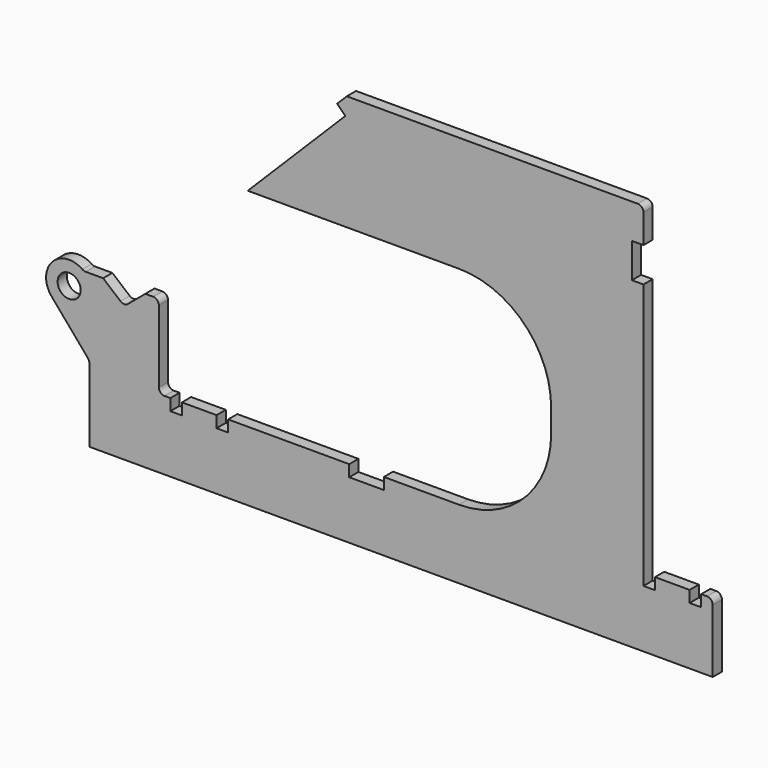
from build123d import *

# Parameters (mm, degrees)
F0_R     = 6.35
F1_DEPTH = 6.35
F2_R     = 3.175
F3_R     = 5.08
F4_R     = 3.175
F5_R     = 3.175


# Not quite as in the source:
# - ends of sketch curves that miss each other by under 0.0002 mm in the source are joined


with BuildPart() as f1:
    # F0 (on Front) → F1 (new body)
    with BuildSketch(Plane.XZ):
        with BuildLine():
            Line((-72.7094654823, -50.272475262), (-83.3648741359, -50.272475262))
            ThreePointArc((-83.3648741359, -50.272475262), (-100.4842470659, -51.222143603), (-101.056400417, -68.3582903151))
            Line((-101.056400417, -68.3582903151), (-80.147210941, -92.8018072064))
            Line((-80.147210941, -92.8018072064), (-80.147210941, -134.409975262))
            Line((-80.147210941, -134.409975262), (262.752789059, -134.409975262))
            Line((262.752789059, -134.409975262), (262.752789059, -96.309975262))
            Line((262.752789059, -96.309975262), (256.402789059, -96.309975262))
            Line((256.402789059, -96.309975262), (256.402789059, -102.659975262))
            Line((256.402789059, -102.659975262), (250.052789059, -102.659975262))
            Line((250.052789059, -102.659975262), (250.052789059, -96.309975262))
            Line((250.052789059, -96.309975262), (231.002789059, -96.309975262))
            Line((231.002789059, -96.309975262), (231.002789059, -102.659975262))
            Line((231.002789059, -102.659975262), (224.652789059, -102.659975262))
            Line((224.652789059, -102.659975262), (224.652789059, 43.390024738))
            Line((224.652789059, 43.390024738), (218.302789059, 43.390024738))
            Line((218.302789059, 43.390024738), (218.302789059, 62.440024738))
            Line((218.302789059, 62.440024738), (224.652789059, 62.440024738))
            Line((224.652789059, 62.440024738), (224.652789059, 81.490024738))
            Line((224.652789059, 81.490024738), (61.4126609984, 81.490024738))
            Line((61.4126609984, 81.490024738), (56.0792184251, 76.1565821646))
            Line((56.0792184251, 76.1565821646), (60.5693464856, 71.6664541041))
            Line((60.5693464856, 71.6664541041), (6.8929171195, 17.990024738))
            Line((6.8929171195, 17.990024738), (123.052789059, 17.990024738))
            ThreePointArc((123.052789059, 17.990024738), (158.9738135432, 3.1110492223), (173.852789059, -32.809975262))
            Line((173.852789059, -32.809975262), (173.852789059, -45.509975262))
            ThreePointArc((173.852789059, -45.509975262), (158.9738135432, -81.4309997463), (123.052789059, -96.309975262))
            Line((123.052789059, -96.309975262), (81.777789059, -96.309975262))
            Line((81.777789059, -96.309975262), (81.777789059, -102.659975262))
            Line((81.777789059, -102.659975262), (62.727789059, -102.659975262))
            Line((62.727789059, -102.659975262), (62.727789059, -96.309975262))
            Line((62.727789059, -96.309975262), (-3.947210941, -96.309975262))
            Line((-3.947210941, -96.309975262), (-3.947210941, -102.659975262))
            Line((-3.947210941, -102.659975262), (-10.297210941, -102.659975262))
            Line((-10.297210941, -102.659975262), (-10.297210941, -96.309975262))
            Line((-10.297210941, -96.309975262), (-29.347210941, -96.309975262))
            Line((-29.347210941, -96.309975262), (-29.347210941, -102.659975262))
            Line((-29.347210941, -102.659975262), (-35.697210941, -102.659975262))
            Line((-35.697210941, -102.659975262), (-35.697210941, -96.309975262))
            Line((-35.697210941, -96.309975262), (-42.047210941, -96.309975262))
            Line((-42.047210941, -96.309975262), (-42.047210941, -50.272475262))
            Line((-42.047210941, -50.272475262), (-49.4849563998, -50.272475262))
            Line((-49.4849563998, -50.272475262), (-61.097210941, -60.0163137647))
            Line((-61.097210941, -60.0163137647), (-72.7094654823, -50.272475262))
        make_face()
        with Locations((-91.4055753496, -60.1028935639)):
            Circle(F0_R, mode=Mode.SUBTRACT)
    extrude(amount=-F1_DEPTH)

    # F2
    f2_edges = [f1.edges().sort_by_distance(p)[0] for p in [
        (224.652789, 3.175, 81.490025),
        (-42.047211, 3.175, -96.309975),
    ]]
    fillet(f2_edges, radius=F2_R)

    # F3
    f3_edges = [f1.edges().sort_by_distance(p)[0] for p in [
        (-80.147211, 3.175, -92.801807),
    ]]
    fillet(f3_edges, radius=F3_R)

    # F4
    f4_edges = [f1.edges().sort_by_distance(p)[0] for p in [
        (-42.047211, 3.175, -50.272475),
    ]]
    fillet(f4_edges, radius=F4_R)

    # F5
    f5_edges = [f1.edges().sort_by_distance(p)[0] for p in [
        (-61.097211, 3.175, -60.016314),
        (-83.364874, 3.175, -50.272475),
        (262.752789, 3.175, -96.309975),
    ]]
    fillet(f5_edges, radius=F5_R)


solid = f1.part
